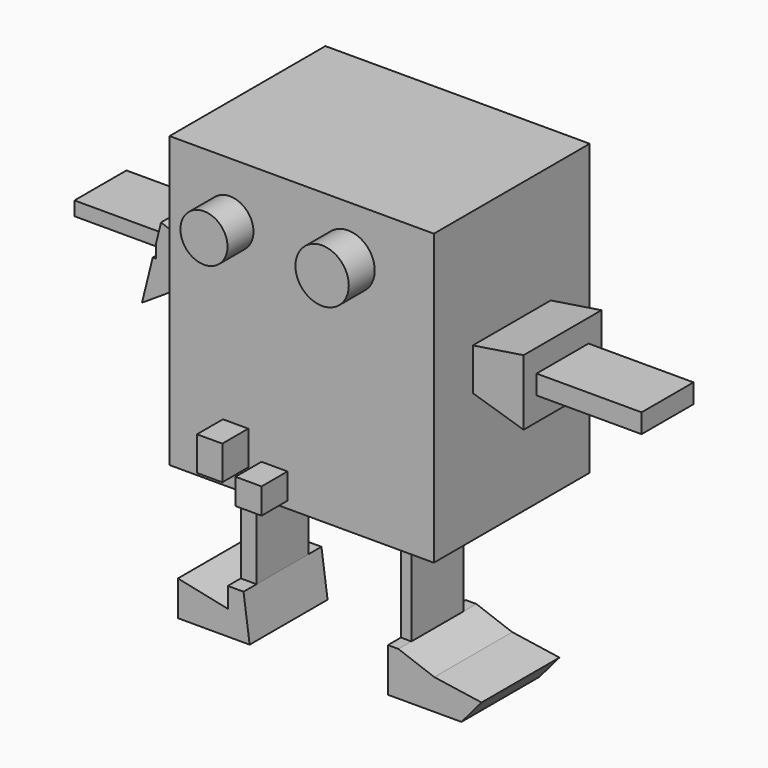
from build123d import *

# Parameters (mm, degrees)
F0_R     = 4.6050240083
F1_DEPTH = 25.4
F0_R_2   = 5.2163960765
F0_W     = 5.0996192879
F0_H     = 5.0427047919
F0_W_2   = 4.9532863107
F0_H_2   = 6.6598858346
F2_DEPTH = 19.05
F0_W_3   = 20.5373242497
F0_H_3   = 3.765176516
F3_DEPTH = 6.35
F0_W_4   = 2.0537329838
F0_H_4   = 23.4467815608
F0_W_5   = 3.08059901
F4_DEPTH = 9.525
F6_DEPTH = 25.4


# Not quite as in the source:
# - the program builds the solid bodies; features that only make, move or delete a surface that nothing else refers to are left out


with BuildPart() as f1:
    # F0 (on Front) → F1 (new body)
    with BuildSketch(Plane.XZ):
        with Locations((-14.0338391066, 17.2000098974)):
            Circle(F0_R)
    extrude(amount=F1_DEPTH)


with BuildPart() as f1b:
    # F0 (on Front) → F1, piece 2 (new body)
    with BuildSketch(Plane.XZ):
        with Locations((9.070652537, 18.2268768549)):
            Circle(F0_R_2)
    extrude(amount=F1_DEPTH)


with BuildPart() as f2:
    # F0 (on Front) → F2 (new body, symmetric)
    with BuildSketch(Plane.XZ):
        Polygon((-25.8428025991, 0), (-25.8428025991, -28.3243972808), (-22.0776256174, -28.3243972808), (-18.9970266074, -28.3243972808), (9.24179703, -28.3243972808), (11.2955300137, -28.3243972808), (25.8428025991, -28.3243972808), (25.8428025991, -2.9950267635), (25.8428025991, 5.2199037746), (25.8428025991, 28.3243972808), (-25.8428025991, 28.3243972808), (-25.8428025991, 3.1661712565), align=None)
        with Locations((-5.3228323739, -24.4338870788)):
            Rectangle(F0_W, F0_H, mode=Mode.SUBTRACT)
        with Locations((-12.9263509633, -20.3735558485)):
            Rectangle(F0_W_2, F0_H_2, mode=Mode.SUBTRACT)
        with Locations((-14.0338391066, 17.2000098974)):
            Circle(F0_R, mode=Mode.SUBTRACT)
        with Locations((9.070652537, 18.2268768549)):
            Circle(F0_R_2, mode=Mode.SUBTRACT)
    extrude(amount=F2_DEPTH, both=True)

    # F0 (on Front) → F3, piece 2 (join, symmetric)
    with BuildSketch(Plane.XZ):
        with Locations((10.2686635219, -40.0477880612)):
            Rectangle(F0_W_4, F0_H_4)
        with Locations((-20.5373261124, -40.0477880612)):
            Rectangle(F0_W_5, F0_H_4)
    extrude(amount=F3_DEPTH, both=True)

    # F0 (on Front) → F6 (join, symmetric)
    with BuildSketch(Plane.XZ):
        with Locations((-12.9263509633, -20.3735558485)):
            Rectangle(F0_W_2, F0_H_2)
        with Locations((-5.3228323739, -24.4338870788)):
            Rectangle(F0_W, F0_H)
    extrude(amount=F6_DEPTH, both=True)


with BuildPart() as f3:
    # F0 (on Front) → F3 (new body, symmetric)
    with BuildSketch(Plane.XZ):
        with Locations((46.0378415883, 0.4278609995)):
            Rectangle(F0_W_3, F0_H_3)
    extrude(amount=F3_DEPTH, both=True)


with BuildPart() as f3b:
    # F0 (on Front) → F3, piece 3 (new body, symmetric)
    with BuildSketch(Plane.XZ):
        Polygon((-54.5950606465, 0), (-36.7501180492, 0), (-36.0735851604, 2.7296595719), (-54.5950606465, 2.7296595719), align=None)
    extrude(amount=F3_DEPTH, both=True)


with BuildPart() as f4:
    # F0 (on Front) → F4 (new body, symmetric)
    with BuildSketch(Plane.XZ):
        Polygon((35.7691794634, 6.7602032796), (25.8428025991, 5.2199037746), (25.8428025991, -2.9950267635), (35.7691794634, -6.0756253079), (35.7691794634, -1.4547272585), (35.7691794634, 2.3104492575), align=None)
    extrude(amount=F4_DEPTH, both=True)


with BuildPart() as f4b:
    # F0 (on Front) → F4, piece 2 (new body, symmetric)
    with BuildSketch(Plane.XZ):
        Polygon((11.2955300137, -51.7711788416), (9.24179703, -51.7711788416), (9.24179703, -60.3283941746), (23.617926985, -60.3283941746), (27.5542456657, -55.7074993849), (18.3124504983, -54.3383434415), align=None)
    extrude(amount=F4_DEPTH, both=True)


with BuildPart() as f4c:
    # F0 (on Front) → F4, piece 3 (new body, symmetric)
    with BuildSketch(Plane.XZ):
        Polygon((-18.9970266074, -51.7711788416), (-22.0776256174, -51.7711788416), (-22.0776256174, -55.7074993849), (-31.8328551948, -53.6537654698), (-31.8328551948, -60.4995377362), (-17.7990160882, -60.4995377362), align=None)
    extrude(amount=F4_DEPTH, both=True)


with BuildPart() as f4d:
    # F0 (on Front) → F4, piece 4 (new body, symmetric)
    with BuildSketch(Plane.XZ):
        Polygon((-38.8497747481, -8.4716472775), (-25.8428025991, 0), (-25.8428025991, 3.1661712565), (-35.1238397671, 6.5616707666), (-36.0735851604, 2.7296595719), (-36.0735851604, 0), (-36.7501180492, 0), align=None)
    extrude(amount=F4_DEPTH, both=True)


solid = Compound([f1.part, f1b.part, f2.part, f3.part, f3b.part, f4.part, f4b.part, f4c.part, f4d.part])
